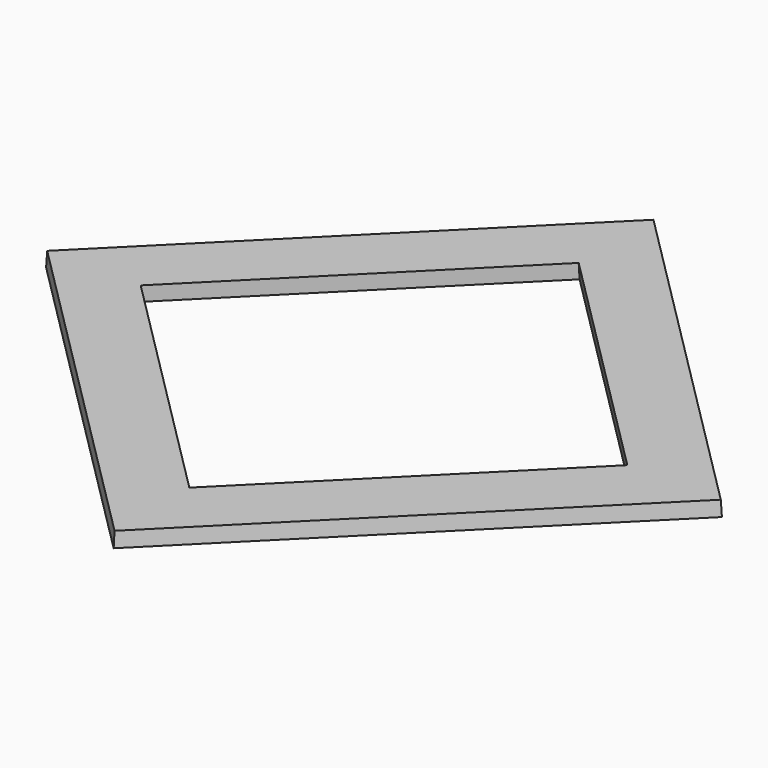
from build123d import *

# Parameters (mm, degrees)
F0_W     = 101.6
F0_H     = 101.6
F1_DEPTH = 3.175
F1_TAPER = 3
F2_T     = -14.0335
F4_ANGLE = 45


# Not quite as in the source:
# - a feature of the source that left no trace in its solid (it failed there, or was rolled back) is left out


with BuildPart() as f1:
    # F0 (on Top) → F1 (new body)
    with BuildSketch(Plane.XY):
        Rectangle(F0_W, F0_H)
    extrude(amount=F1_DEPTH, taper=F1_TAPER)

    # F2
    f2_openings = [f1.faces().sort_by_distance(p)[0] for p in [
        (0, 0, 3.175),
        (0, 0, 0),
    ]]
    offset(amount=F2_T, openings=f2_openings)


with BuildPart() as f1_1:
    # F4: moved
    add(f1.part.rotate(Axis((0, 0, 69.4056898355), (0, 0, 1)), F4_ANGLE))


solid = f1_1.part
